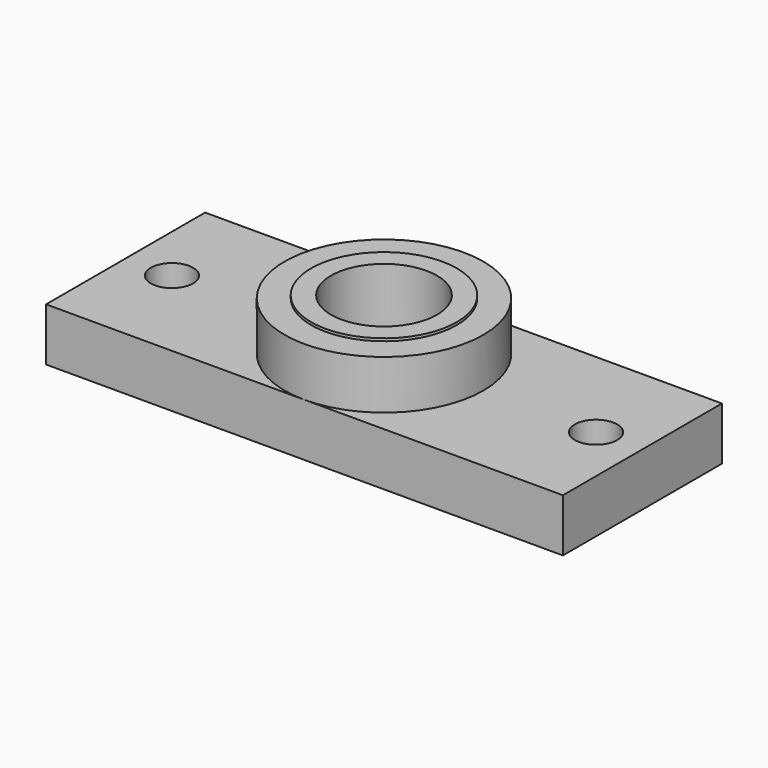
from build123d import *

# Parameters (mm, degrees)
F0_W      = 39
F0_H      = 15
F1_DEPTH  = 4
F2_R      = 7.5
F3_DEPTH  = 3.9
F4_R      = 4
F5_DEPTH  = 4.2
F6_R      = 1.6
F7_DEPTH  = 25
F8_R      = 1.45
F9_DEPTH  = 25
F10_R     = 7.5
F10_R_2   = 5.5
F11_DEPTH = 0.2


# Not quite as in the source:
# - a feature names something its author has since deleted; it is built from what else it names


with BuildPart() as f1:
    # F0 (on Top) → F1 (new body)
    with BuildSketch(Plane.XY):
        with Locations((19.5, 7.5)):
            Rectangle(F0_W, F0_H)
    extrude(amount=F1_DEPTH)

    # F2 (on face) → F3 (join)
    with BuildSketch(Plane.XY.offset(4)):
        with Locations((19.5, 7.5)):
            Circle(F2_R)
    extrude(amount=F3_DEPTH)

    # F4 (on face) → F5 (cut)
    with BuildSketch(Plane.XY.offset(7.9)):
        with Locations((19.5, 7.5)):
            Circle(F4_R)
    extrude(amount=-F5_DEPTH, mode=Mode.SUBTRACT)

    # F6 (on face) → F7 (cut)
    with BuildSketch(Plane.XY.offset(4)):
        with Locations((35.5, 7.5)):
            Circle(F6_R)
        with Locations((3.5, 7.5)):
            Circle(F6_R)
    extrude(amount=-F7_DEPTH, mode=Mode.SUBTRACT)

    # F8 (on face) → F9 (cut)
    with BuildSketch(Plane.XY.offset(3.7)):
        with Locations((19.5, 7.5)):
            Circle(F8_R)
    extrude(amount=-F9_DEPTH, mode=Mode.SUBTRACT)

    # F10 (on face) → F11 (cut)
    with BuildSketch(Plane.XY.offset(7.9)):
        with Locations((19.5, 7.5)):
            Circle(F10_R)
        with Locations((19.5, 7.5)):
            Circle(F10_R_2, mode=Mode.SUBTRACT)
    extrude(amount=-F11_DEPTH, mode=Mode.SUBTRACT)


solid = f1.part
